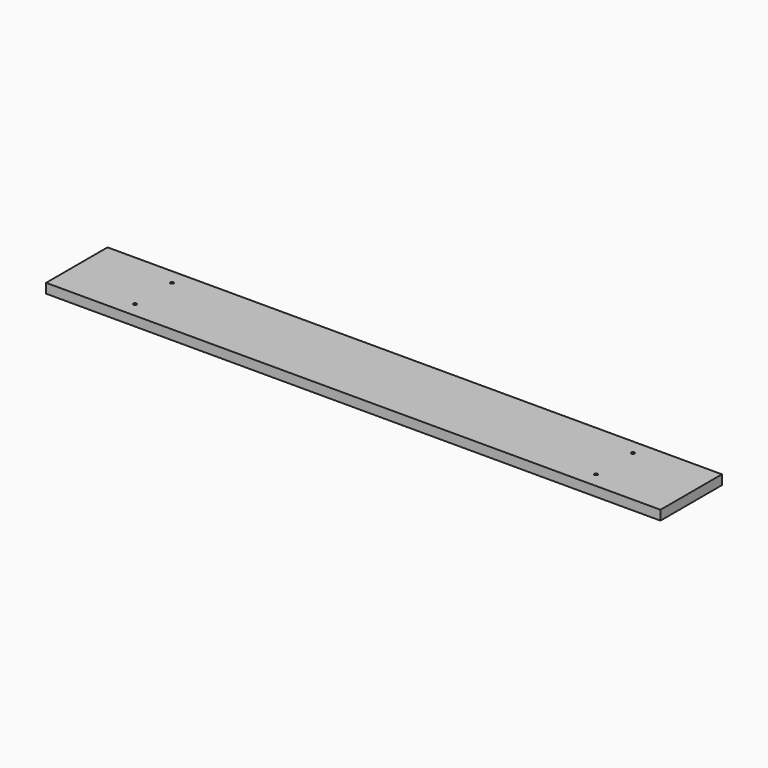
from build123d import *

# Parameters (mm, degrees)
F1_W     = 1219.2
F1_H     = 152.4
F1_R     = 3.175
F2_DEPTH = 19.05


# Not quite as in the source:
# - a variable given as a bare number and used for a length is read in inches; the dataset says mm whatever the document's units were


with BuildPart() as f2:
    # F1 (on Top) → F2 (new body)
    with BuildSketch(Plane.XY):
        Rectangle(F1_W, F1_H)
        with Locations((-457.2, -45.72)):
            Circle(F1_R, mode=Mode.SUBTRACT)
        with Locations((457.2, -45.72)):
            Circle(F1_R, mode=Mode.SUBTRACT)
        with Locations((-457.2, 45.72)):
            Circle(F1_R, mode=Mode.SUBTRACT)
        with Locations((457.2, 45.72)):
            Circle(F1_R, mode=Mode.SUBTRACT)
    extrude(amount=F2_DEPTH)


solid = f2.part
